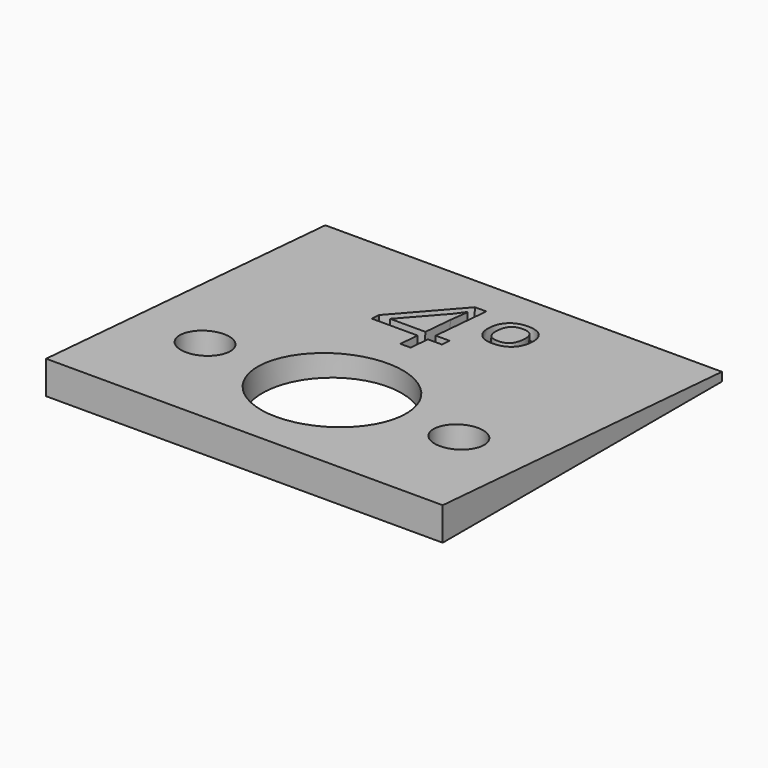
from build123d import *

# Parameters (mm, degrees)
F1_DEPTH     = 12.5
F2_R         = 1.5
F2_R_2       = 4.4
F3_DEPTH     = 25
F4_TEXT_SIZE = 8.3333333333
F5_DEPTH     = 25


# Not quite as in the source:
# - Text() gives the source's letters only with a copy of the font that has no kerning and outlines rounded to 1/6400 em; it was checked with that copy


with BuildPart() as f1:
    # F0 (on Right) → F1 (new body, symmetric)
    with BuildSketch(Plane.YZ):
        Polygon((0, 0), (22, 0), (22, 0.5441051397), (0, 2.0824950024), align=None)
    extrude(amount=F1_DEPTH, both=True)

    # F2 (on Top) → F3 (cut)
    with BuildSketch(Plane.XY):
        with Locations((8, 6.9)):
            Circle(F2_R)
        with Locations((-8, 6.9)):
            Circle(F2_R)
        with Locations((0, 6.9)):
            Circle(F2_R_2)
    extrude(amount=F3_DEPTH, mode=Mode.SUBTRACT)

    # F4 (on face) → F5 (cut)
    with BuildSketch(Plane(origin=(0, 0.1449136436, 2.0723616533), x_dir=(1, 0, 0), z_dir=(0, 0.0697564737, 0.9975640503))):
        with Locations((-4.0807291667, 13.4400025747)):
            Text('4º', F4_TEXT_SIZE, font='Open Sans', text_align=(TextAlign.LEFT, TextAlign.BOTTOM))
    extrude(amount=-F5_DEPTH, mode=Mode.SUBTRACT)


solid = f1.part
